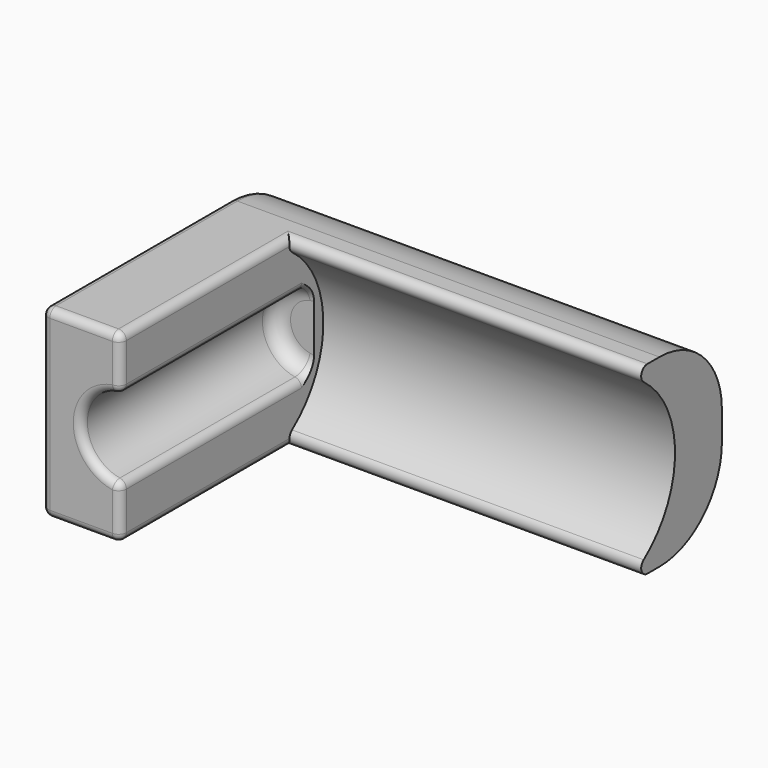
from build123d import *

# Parameters (mm, degrees)
F0_W          = 13.97
F0_H          = 5.08
F1_DEPTH      = 6
F3_DEPTH      = 5.08
F4_R          = 3.175
F5_DEPTH      = 11.43
F6_R          = 1.27
F7_DEPTH      = 7.874
F8_R          = 2.54
F9_R          = 0.254
F10_T2_ANGLE  = 160.8118635463
F10_T6_ANGLE  = 359.64
F10_T11_ANGLE = 359.64


# Not quite as in the source:
# - a fillet or chamfer that OpenCascade refuses, or shapes differently, is made with other operations: its cross-section is extruded or revolved along the edge and cut away or added


with BuildPart() as f1:
    # F0 (on Top) → F1 (new body)
    with BuildSketch(Plane.XY):
        with Locations((-6.985, -2.54)):
            Rectangle(F0_W, F0_H)
    extrude(amount=F1_DEPTH)

    # F2 (on face) → F3 (join)
    with BuildSketch(Plane.XZ.offset(5.08)):
        Polygon((-11.43, 6), (-13.97, 6), (-13.97, 0), (-11.43, 0), (-11.43, 1.7556592107), align=None)
    extrude(amount=F3_DEPTH)

    # F4 (on face) → F5 (cut)
    with BuildSketch(Plane.YZ):
        with Locations((-5.08, 3)):
            Circle(F4_R)
    extrude(amount=-F5_DEPTH, mode=Mode.SUBTRACT)

    # F6 (on face) → F7 (cut)
    with BuildSketch(Plane.XZ.offset(10.16)):
        with Locations((-11.43, 3)):
            Circle(F6_R)
    extrude(amount=-F7_DEPTH, mode=Mode.SUBTRACT)

    # F8
    f8_edges = [f1.edges().sort_by_distance(p)[0] for p in [
        (-6.985, 0, 6),
        (-6.985, 0, 0),
    ]]
    fillet(f8_edges, radius=F8_R)

    # F9
    f9_edges = [f1.edges().sort_by_distance(p)[0] for p in [
        (-11.43, -10.16, 5.135),
        (-12.7, -10.16, 6),
        (-12.7, -10.16, 3),
        (-11.43, -10.16, 0.865),
        (-12.7, -10.16, 0),
        (-13.97, -10.16, 3),
        (-13.97, -6.35, 6),
        (-11.43, -7.100234, 6),
        (-11.43, -7.100234, 0),
        (-11.43, -6.223, 1.73),
        (-11.43, -6.223, 4.27),
        (-5.715, -4.040469, 6),
        (-5.715, -4.040469, 0),
        (-13.97, -6.35, 0),
        (-13.97, -0.743949, 0.743949),
        (-13.97, 0, 3),
        (-13.97, -0.743949, 5.256051),
    ]]
    fillet(f9_edges, radius=F9_R)

    # F10: fillet of radius 0.508 on 1 edges, made by hand

    # F10_s1 → F10_t2 (revolve)
    with BuildSketch(Plane(origin=(-10.6194933514, 0, -1.7950219978), x_dir=(0, 1, 0), z_dir=(0.9860132972, 0, 0.1666666667))):
        with BuildLine():
            ThreePointArc((-2.286, 5.6250398915), (-2.4347897552, 5.9842501364), (-2.794, 6.1330398915))
            Line((-2.794, 6.1330398915), (-2.286, 6.1330398915))
            Line((-2.286, 6.1330398915), (-2.286, 5.6250398915))
        make_face()
    revolve(axis=Axis((-11.43, -2.286, 3), (0, -1, 0)), revolution_arc=F10_T2_ANGLE)


with BuildPart() as f10_tool4:
    # F10_s5 → F10_t6 (revolve)
    with BuildSketch(Plane(origin=(-10.6699629137, 0, -1.7346683419), x_dir=(0, 1, 0), z_dir=(0.9870410248, 0, 0.1604681133))):
        with BuildLine():
            ThreePointArc((-2.794, 6.065243527), (-2.4347897552, 5.9164537719), (-2.286, 5.557243527))
            Line((-2.286, 5.557243527), (-2.286, 6.065243527))
            Line((-2.286, 6.065243527), (-2.794, 6.065243527))
        make_face()
    revolve(axis=Axis((-11.684, -2.286, 4.5026842649), (0, 1, 0)), revolution_arc=F10_T6_ANGLE)

    split(bisect_by=Plane.YZ.offset(-11.43), keep=Keep.BOTTOM)


with BuildPart() as f1_1:
    add(f1.part)

    # F10_t3: union F10_tool4
    add(f10_tool4.part)


with BuildPart() as f10_tool9:
    # F10_s10 → F10_t11 (revolve)
    with BuildSketch(Plane(origin=(-11.6202945797, 0, 1.8891684342), x_dir=(0, 1, 0), z_dir=(0.9870410248, 0, -0.1604681133))):
        with BuildLine():
            ThreePointArc((-2.794, -0.1429973783), (-2.4347897552, 0.0057923768), (-2.286, 0.3650026217))
            Line((-2.286, 0.3650026217), (-2.286, -0.1429973783))
            Line((-2.286, -0.1429973783), (-2.794, -0.1429973783))
        make_face()
    revolve(axis=Axis((-11.684, -2.286, 1.4973157351), (0, -1, 0)), revolution_arc=F10_T11_ANGLE)

    split(bisect_by=Plane.YZ.offset(-11.43), keep=Keep.BOTTOM)


with BuildPart() as f1_2:
    add(f1_1.part)

    # F10_t8: union F10_tool9
    add(f10_tool9.part)


solid = f1_2.part
